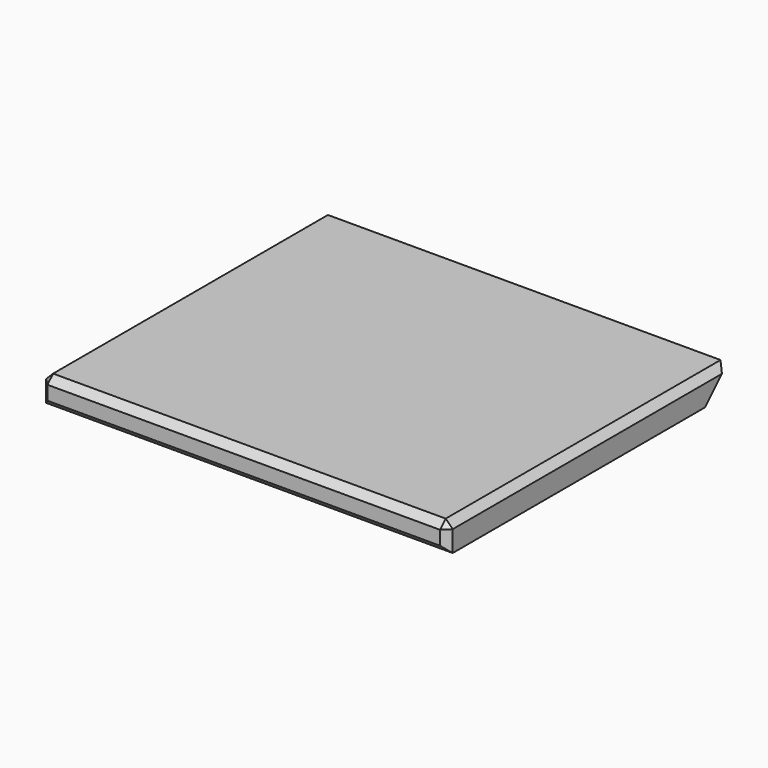
from build123d import *

# Parameters (mm, degrees)
F0_W     = 290
F0_H     = 250
F1_DEPTH = 20
F2_SIZE  = 19.99999
F3_SIZE  = 5


# Not quite as in the source:
# - a fillet or chamfer is up to 0.001 mm smaller than in the source, because OpenCascade refuses the exact size


with BuildPart() as f1:
    # F0 (on Top) → F1 (new body)
    with BuildSketch(Plane.XY):
        Rectangle(F0_W, F0_H)
    extrude(amount=F1_DEPTH)

    # F2 (size 20 in the source; OpenCascade refuses exactly that, so slightly less here)
    f2_edges = [f1.edges().sort_by_distance(p)[0] for p in [
        (0, 125, 0),
    ]]
    chamfer(f2_edges, length=F2_SIZE)

    # F3
    f3_edges = [f1.edges().sort_by_distance(p)[0] for p in [
        (0, -125, 20),
        (0, -125, 0),
        (145, 0, 20),
        (145, -125, 10),
        (-145, -125, 10),
        (-145, 0, 20),
    ]]
    chamfer(f3_edges, length=F3_SIZE)


solid = f1.part
